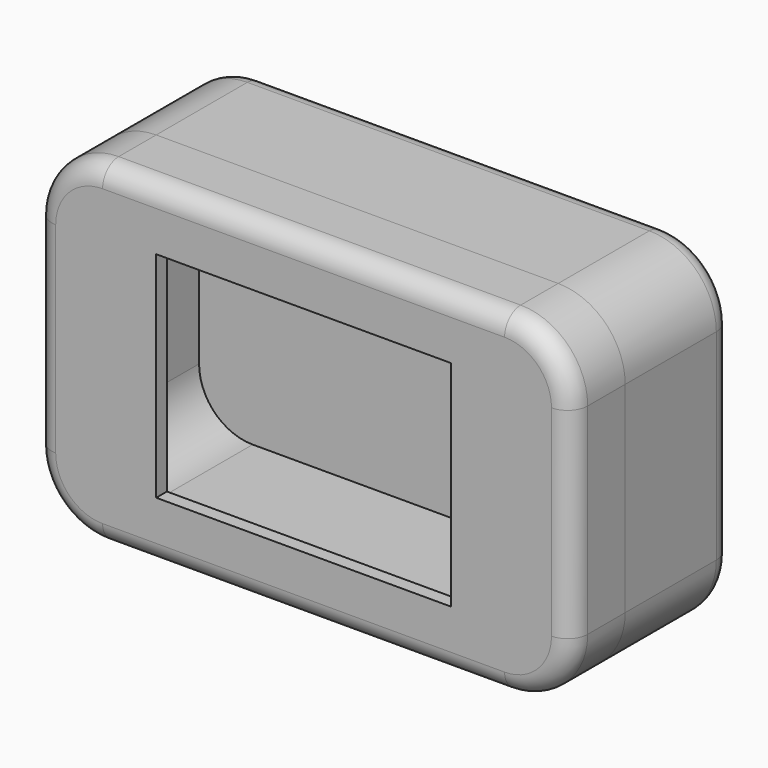
from build123d import *

# Parameters (mm, degrees)
F1_DEPTH = 12.7
F3_DEPTH = 25.4
F4_T     = -2.54
F4_2_T   = -2.54
F2_W     = 55.88
F2_H     = 40.64
F5_DEPTH = 38.101
F6_R     = 3.81
F6_2_R   = 3.81


with BuildPart() as f1:
    # F0 (on Front) → F1 (new body)
    with BuildSketch(Plane.XZ):
        with BuildLine():
            Line((-38.1, -31.75), (38.1, -31.75))
            ThreePointArc((38.1, -31.75), (47.0802561211, -28.0302561211), (50.8, -19.05))
            Line((50.8, -19.05), (50.8, 19.05))
            ThreePointArc((50.8, 19.05), (47.0802561211, 28.0302561211), (38.1, 31.75))
            Line((38.1, 31.75), (-38.1, 31.75))
            ThreePointArc((-38.1, 31.75), (-47.0802561211, 28.0302561211), (-50.8, 19.05))
            Line((-50.8, 19.05), (-50.8, -19.05))
            ThreePointArc((-50.8, -19.05), (-47.0802561211, -28.0302561211), (-38.1, -31.75))
        make_face()
    extrude(amount=F1_DEPTH)

    # F4
    f4_openings = [f1.faces().sort_by_distance(p)[0] for p in [
        (0, 0, 0),
    ]]
    offset(amount=F4_T, openings=f4_openings)

    # F2 (on face) → F5 (cut, through all)
    with BuildSketch(Plane.XZ.offset(12.7)):
        Rectangle(F2_W, F2_H)
    extrude(amount=-F5_DEPTH, mode=Mode.SUBTRACT)

    # F6
    f6_edges = [f1.edges().sort_by_distance(p)[0] for p in [
        (0, -12.7, 31.75),
        (0, -12.7, -31.75),
        (-47.080256, -12.7, -28.030256),
        (47.080256, -12.7, -28.030256),
        (-50.8, -12.7, 0),
        (50.8, -12.7, 0),
        (-47.080256, -12.7, 28.030256),
        (47.080256, -12.7, 28.030256),
    ]]
    fillet(f6_edges, radius=F6_R)


with BuildPart() as f3:
    # F0 (on Front) → F3 (new body)
    with BuildSketch(Plane.XZ):
        with BuildLine():
            Line((-38.1, -31.75), (38.1, -31.75))
            ThreePointArc((38.1, -31.75), (47.0802561211, -28.0302561211), (50.8, -19.05))
            Line((50.8, -19.05), (50.8, 19.05))
            ThreePointArc((50.8, 19.05), (47.0802561211, 28.0302561211), (38.1, 31.75))
            Line((38.1, 31.75), (-38.1, 31.75))
            ThreePointArc((-38.1, 31.75), (-47.0802561211, 28.0302561211), (-50.8, 19.05))
            Line((-50.8, 19.05), (-50.8, -19.05))
            ThreePointArc((-50.8, -19.05), (-47.0802561211, -28.0302561211), (-38.1, -31.75))
        make_face()
    extrude(amount=-F3_DEPTH)

    # F4#2
    f4_2_openings = [f3.faces().sort_by_distance(p)[0] for p in [
        (0, 0, 0),
    ]]
    offset(amount=F4_2_T, openings=f4_2_openings)

    # F6#2
    f6_2_edges = [f3.edges().sort_by_distance(p)[0] for p in [
        (0, 25.4, 31.75),
        (0, 25.4, -31.75),
        (47.080256, 25.4, -28.030256),
        (50.8, 25.4, 0),
        (47.080256, 25.4, 28.030256),
        (-47.080256, 25.4, 28.030256),
        (-50.8, 25.4, 0),
        (-47.080256, 25.4, -28.030256),
    ]]
    fillet(f6_2_edges, radius=F6_2_R)


solid = Compound([f1.part, f3.part])
